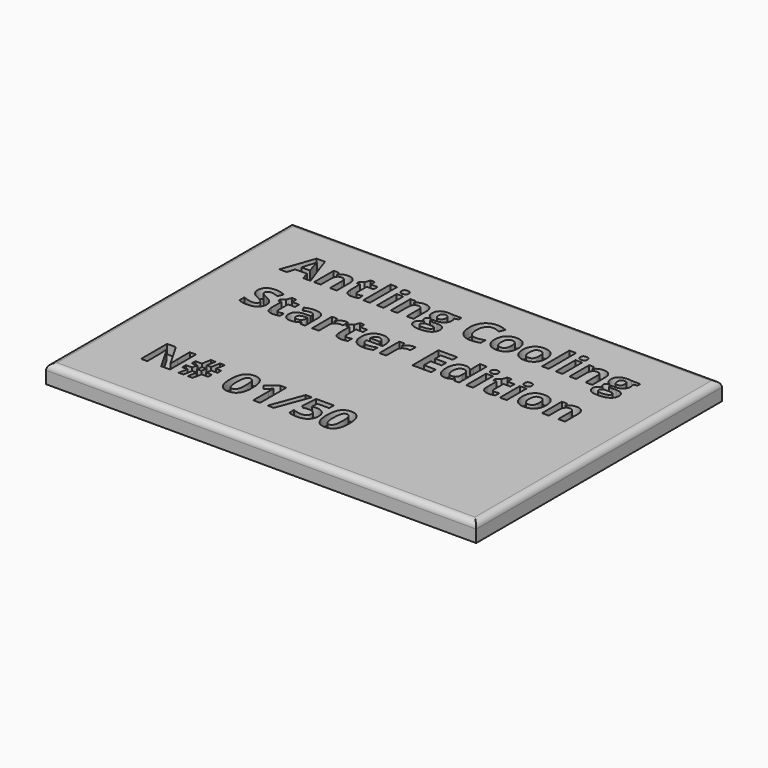
from build123d import *

# Parameters (mm, degrees)
F0_W         = 70
F0_H         = 50
F1_DEPTH     = 3
F2_R         = 1
F3_TEXT_SIZE = 7.3347931973
F4_DEPTH     = 1.5
F5_TEXT_SIZE = 7.4124914207
F6_DEPTH     = 1.5


# Not quite as in the source:
# - Text() gives the source's letters only with a copy of the font that has no kerning and outlines rounded to 1/6400 em; it was checked with that copy


with BuildPart() as f1:
    # F0 (on Top) → F1 (new body)
    with BuildSketch(Plane.XY):
        with Locations((1.6883611679, 3.3117169408)):
            Rectangle(F0_W, F0_H)
    extrude(amount=F1_DEPTH)

    # F2
    f2_edges = [f1.edges().sort_by_distance(p)[0] for p in [
        (-33.311639, 3.311717, 3),
        (1.688361, 28.311717, 3),
        (1.688361, -21.688283, 3),
        (36.688361, 3.311717, 3),
    ]]
    fillet(f2_edges, radius=F2_R)

    # F3 (on face) → F4 (cut)
    with BuildSketch(Plane.XY.offset(3)):
        with Locations((-26.3116388321, 17.0306658388)):
            Text('Antling Cooling', F3_TEXT_SIZE, font='Open Sans', font_style=FontStyle.BOLD, text_align=(TextAlign.LEFT, TextAlign.BOTTOM))
    extrude(amount=-F4_DEPTH, mode=Mode.SUBTRACT)

    # F5 (on face) → F6 (cut)
    with BuildSketch(Plane.XY.offset(3)):
        with Locations((-25.3116388321, 6.9747231179)):
            Text('Starter Edition', F5_TEXT_SIZE, font='Open Sans', font_style=FontStyle.BOLD, text_align=(TextAlign.LEFT, TextAlign.BOTTOM))
        with Locations((-25.3116388321, -13.1872535465)):
            Text('N# 01/50', F5_TEXT_SIZE, font='Open Sans', font_style=FontStyle.BOLD, text_align=(TextAlign.LEFT, TextAlign.BOTTOM))
    extrude(amount=-F6_DEPTH, mode=Mode.SUBTRACT)


solid = f1.part
